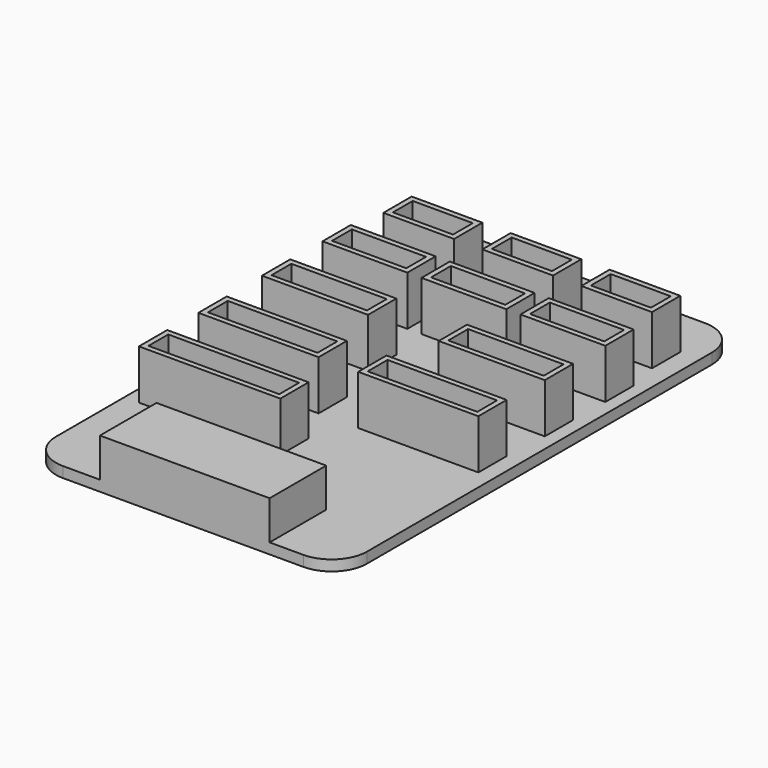
from build123d import *

# Parameters (mm, degrees)
F0_W         = 44
F0_H         = 71
F1_DEPTH     = 1.5
F2_R         = 5
F3_W         = 24
F3_H         = 10
F4_DEPTH     = 5.5
F5_W         = 10
F5_H         = 5
F5_W_2       = 12
F5_W_3       = 15
F5_W_4       = 17
F5_W_5       = 20
F6_DEPTH     = 7
F7_T         = 0.75
F7_T3_DEPTH  = 11.5
F7_T5_DEPTH  = 25.5
F7_T7_DEPTH  = 6.5
F7_T9_DEPTH  = 21.5
F7_T11_DEPTH = 6.5
F7_T13_DEPTH = 18.5
F7_T15_DEPTH = 18.5
F7_T17_DEPTH = 6.5
F7_T19_DEPTH = 16.5
F7_T21_DEPTH = 6.5
F7_T23_DEPTH = 13.5
F7_T25_DEPTH = 11.5
F7_T27_DEPTH = 6.5
F7_T29_DEPTH = 13.5
F7_T31_DEPTH = 16.5
F7_T33_DEPTH = 13.5
F7_T35_DEPTH = 11.5
F7_T37_DEPTH = 11.5


# Not quite as in the source:
# - a shell that OpenCascade refuses in one call is made with other operations: the cavity is built on its own and cut out


with BuildPart() as f1:
    # F0 (on Top) → F1 (new body)
    with BuildSketch(Plane.XY):
        with Locations((-0.4986094981, 2.3689430654)):
            Rectangle(F0_W, F0_H)
    extrude(amount=F1_DEPTH)

    # F2
    f2_edges = [f1.edges().sort_by_distance(p)[0] for p in [
        (-22.498609, 37.868943, 0.75),
        (-22.498609, -33.131057, 0.75),
        (21.501391, -33.131057, 0.75),
        (21.501391, 37.868943, 0.75),
    ]]
    fillet(f2_edges, radius=F2_R)

    # F3 (on face) → F4 (join)
    with BuildSketch(Plane.XY.offset(1.5)):
        with Locations((-0.276770547, -28.1310569346)):
            Rectangle(F3_W, F3_H)
    extrude(amount=F4_DEPTH)

    # F5 (on face) → F6 (join)
    with BuildSketch(Plane.XY.offset(1.5)):
        with Locations((-14.3074645847, 28.2659181952)):
            Rectangle(F5_W, F5_H)
        with Locations((-0.3074645847, 28.2659181952)):
            Rectangle(F5_W, F5_H)
        with Locations((13.6925354153, 28.2659181952)):
            Rectangle(F5_W, F5_H)
        with Locations((-14.3036200255, 18.7520762533)):
            Rectangle(F5_W_2, F5_H)
        with Locations((-0.3036200255, 18.7520762533)):
            Rectangle(F5_W_2, F5_H)
        with Locations((-12.8887149692, 8.1576090865)):
            Rectangle(F5_W_3, F5_H)
        with Locations((-11.8254707158, -3.1629925966)):
            Rectangle(F5_W_4, F5_H)
        with Locations((-10.4394350369, -13.5349402577)):
            Rectangle(F5_W_5, F5_H)
        with Locations((13.6963799745, 18.7520762533)):
            Rectangle(F5_W_2, F5_H)
        with Locations((12.1112850308, 8.1576090865)):
            Rectangle(F5_W_3, F5_H)
        with Locations((10.7745292842, -3.1629925966)):
            Rectangle(F5_W_4, F5_H)
    extrude(amount=F6_DEPTH)

    # F7: shell of thickness 0.75, made by hand


with BuildPart() as f7_core1:
    # F7_t2: copy of F1
    add(f1.part)

    # the walls: a layer under each face that stays
    f7_faces = [f7_core1.faces().sort_by_distance(p)[0] for p in [
        (-0.4986094981, -33.1310569346, 3.5),
        (-0.4986094981, 2.3689430654, 0),
        (-21.0341434041, -31.6665908405, 0.75),
        (-0.4986094981, 2.3689430654, 1.5),
        (-12.276770547, -28.1310569346, 4.25),
        (-0.276770547, -28.1310569346, 7),
        (11.723229453, -28.1310569346, 4.25),
        (20.0369244078, -31.6665908405, 0.75),
        (-22.4986094981, 2.3689430654, 0.75),
        (21.5013905019, 2.3689430654, 0.75),
        (-21.0341434041, 36.4044769713, 0.75),
        (20.0369244078, 36.4044769713, 0.75),
        (-0.4986094981, 37.8689430654, 0.75),
        (-0.276770547, -23.1310569346, 4.25),
        (-20.4394350369, -13.5349402577, 5),
        (-10.4394350369, -16.0349402577, 5),
        (-0.4394350369, -13.5349402577, 5),
        (-10.4394350369, -11.0349402577, 5),
        (-3.3254707158, -3.1629925966, 5),
        (-11.8254707158, -0.6629925966, 5),
        (-20.3254707158, -3.1629925966, 5),
        (-11.8254707158, -5.6629925966, 5),
        (19.2745292842, -3.1629925966, 5),
        (10.7745292842, -0.6629925966, 5),
        (2.2745292842, -3.1629925966, 5),
        (10.7745292842, -5.6629925966, 5),
        (-20.3887149692, 8.1576090865, 5),
        (-12.8887149692, 5.6576090865, 5),
        (-5.3887149692, 8.1576090865, 5),
        (-12.8887149692, 10.6576090865, 5),
        (-20.3036200255, 18.7520762533, 5),
        (-14.3036200255, 16.2520762533, 5),
        (-8.3036200255, 18.7520762533, 5),
        (-14.3036200255, 21.2520762533, 5),
        (-14.3074645847, 30.7659181952, 5),
        (-19.3074645847, 28.2659181952, 5),
        (-14.3074645847, 25.7659181952, 5),
        (-9.3074645847, 28.2659181952, 5),
        (-0.3036200255, 16.2520762533, 5),
        (5.6963799745, 18.7520762533, 5),
        (-0.3036200255, 21.2520762533, 5),
        (-6.3036200255, 18.7520762533, 5),
        (19.6112850308, 8.1576090865, 5),
        (12.1112850308, 10.6576090865, 5),
        (4.6112850308, 8.1576090865, 5),
        (12.1112850308, 5.6576090865, 5),
        (7.6963799745, 18.7520762533, 5),
        (13.6963799745, 16.2520762533, 5),
        (19.6963799745, 18.7520762533, 5),
        (13.6963799745, 21.2520762533, 5),
        (-0.3074645847, 25.7659181952, 5),
        (4.6925354153, 28.2659181952, 5),
        (-0.3074645847, 30.7659181952, 5),
        (-5.3074645847, 28.2659181952, 5),
        (13.6925354153, 30.7659181952, 5),
        (8.6925354153, 28.2659181952, 5),
        (13.6925354153, 25.7659181952, 5),
        (18.6925354153, 28.2659181952, 5),
    ]]
    thicken(f7_faces, amount=-F7_T, mode=Mode.SUBTRACT)

    # F7_s4 → F7_t3 (cut)
    with BuildSketch(Plane.XZ.offset(22.3810569346)):
        Polygon((-12.284270547, 1.5075), (-12.276770547, 0.75), (-11.526770547, 0.75), (-11.526770547, 1.5), align=None)
        Polygon((11.730729453, 1.5075), (11.723229453, 0.75), (10.973229453, 0.75), (10.973229453, 1.5), align=None)
    extrude(amount=F7_T3_DEPTH, mode=Mode.SUBTRACT)

    # F7_s6 → F7_t5 (cut)
    with BuildSketch(Plane.YZ.offset(-13.026770547)):
        Polygon((-23.1235569346, 1.5075), (-23.1310569346, 0.75), (-23.8810569346, 0.75), (-23.8810569346, 1.5), align=None)
    extrude(amount=F7_T5_DEPTH, mode=Mode.SUBTRACT)

    # F7_s8 → F7_t7 (cut)
    with BuildSketch(Plane.XZ.offset(10.2849402577)):
        Polygon((-20.4469350369, 1.5075), (-20.4394350369, 0.75), (-19.6894350369, 0.75), (-19.6894350369, 1.5), align=None)
        Polygon((-0.4319350369, 1.5075), (-0.4394350369, 0.75), (-1.1894350369, 0.75), (-1.1894350369, 1.5), align=None)
    extrude(amount=F7_T7_DEPTH, mode=Mode.SUBTRACT)

    # F7_s10 → F7_t9 (cut)
    with BuildSketch(Plane.YZ.offset(-21.1894350369)):
        Polygon((-16.0424402577, 1.5075), (-16.0349402577, 0.75), (-15.2849402577, 0.75), (-15.2849402577, 1.5), align=None)
        Polygon((-11.0274402577, 1.5075), (-11.0349402577, 0.75), (-11.7849402577, 0.75), (-11.7849402577, 1.5), align=None)
    extrude(amount=F7_T9_DEPTH, mode=Mode.SUBTRACT)

    # F7_s12 → F7_t11 (cut)
    with BuildSketch(Plane.XZ.offset(-0.0870074034)):
        Polygon((-3.3179707158, 1.5075), (-3.3254707158, 0.75), (-4.0754707158, 0.75), (-4.0754707158, 1.5), align=None)
        Polygon((-20.3329707158, 1.5075), (-20.3254707158, 0.75), (-19.5754707158, 0.75), (-19.5754707158, 1.5), align=None)
        Polygon((19.2820292842, 1.5075), (19.2745292842, 0.75), (18.5245292842, 0.75), (18.5245292842, 1.5), align=None)
        Polygon((2.2670292842, 1.5075), (2.2745292842, 0.75), (3.0245292842, 0.75), (3.0245292842, 1.5), align=None)
    extrude(amount=F7_T11_DEPTH, mode=Mode.SUBTRACT)

    # F7_s14 → F7_t13 (cut)
    with BuildSketch(Plane.YZ.offset(-21.0754707158)):
        Polygon((-0.6554925966, 1.5075), (-0.6629925966, 0.75), (-1.4129925966, 0.75), (-1.4129925966, 1.5), align=None)
        Polygon((-5.6704925966, 1.5075), (-5.6629925966, 0.75), (-4.9129925966, 0.75), (-4.9129925966, 1.5), align=None)
    extrude(amount=F7_T13_DEPTH, mode=Mode.SUBTRACT)

    # F7_s16 → F7_t15 (cut)
    with BuildSketch(Plane.YZ.offset(1.5245292842)):
        Polygon((-0.6554925966, 1.5075), (-0.6629925966, 0.75), (-1.4129925966, 0.75), (-1.4129925966, 1.5), align=None)
        Polygon((-5.6704925966, 1.5075), (-5.6629925966, 0.75), (-4.9129925966, 0.75), (-4.9129925966, 1.5), align=None)
    extrude(amount=F7_T15_DEPTH, mode=Mode.SUBTRACT)

    # F7_s18 → F7_t17 (cut)
    with BuildSketch(Plane.XZ.offset(-11.4076090865)):
        Polygon((-20.3962149692, 1.5075), (-20.3887149692, 0.75), (-19.6387149692, 0.75), (-19.6387149692, 1.5), align=None)
        Polygon((-5.3812149692, 1.5075), (-5.3887149692, 0.75), (-6.1387149692, 0.75), (-6.1387149692, 1.5), align=None)
        Polygon((19.6187850308, 1.5075), (19.6112850308, 0.75), (18.8612850308, 0.75), (18.8612850308, 1.5), align=None)
        Polygon((4.6037850308, 1.5075), (4.6112850308, 0.75), (5.3612850308, 0.75), (5.3612850308, 1.5), align=None)
    extrude(amount=F7_T17_DEPTH, mode=Mode.SUBTRACT)

    # F7_s20 → F7_t19 (cut)
    with BuildSketch(Plane.YZ.offset(-21.1387149692)):
        Polygon((5.6501090865, 1.5075), (5.6576090865, 0.75), (6.4076090865, 0.75), (6.4076090865, 1.5), align=None)
        Polygon((10.6651090865, 1.5075), (10.6576090865, 0.75), (9.9076090865, 0.75), (9.9076090865, 1.5), align=None)
    extrude(amount=F7_T19_DEPTH, mode=Mode.SUBTRACT)

    # F7_s22 → F7_t21 (cut)
    with BuildSketch(Plane.XZ.offset(-22.0020762533)):
        Polygon((-20.3111200255, 1.5075), (-20.3036200255, 0.75), (-19.5536200255, 0.75), (-19.5536200255, 1.5), align=None)
        Polygon((-8.2961200255, 1.5075), (-8.3036200255, 0.75), (-9.0536200255, 0.75), (-9.0536200255, 1.5), align=None)
        Polygon((5.7038799745, 1.5075), (5.6963799745, 0.75), (4.9463799745, 0.75), (4.9463799745, 1.5), align=None)
        Polygon((-6.3111200255, 1.5075), (-6.3036200255, 0.75), (-5.5536200255, 0.75), (-5.5536200255, 1.5), align=None)
        Polygon((7.6888799745, 1.5075), (7.6963799745, 0.75), (8.4463799745, 0.75), (8.4463799745, 1.5), align=None)
        Polygon((19.7038799745, 1.5075), (19.6963799745, 0.75), (18.9463799745, 0.75), (18.9463799745, 1.5), align=None)
    extrude(amount=F7_T21_DEPTH, mode=Mode.SUBTRACT)

    # F7_s24 → F7_t23 (cut)
    with BuildSketch(Plane.YZ.offset(-21.0536200255)):
        Polygon((16.2445762533, 1.5075), (16.2520762533, 0.75), (17.0020762533, 0.75), (17.0020762533, 1.5), align=None)
        Polygon((21.2595762533, 1.5075), (21.2520762533, 0.75), (20.5020762533, 0.75), (20.5020762533, 1.5), align=None)
    extrude(amount=F7_T23_DEPTH, mode=Mode.SUBTRACT)

    # F7_s26 → F7_t25 (cut)
    with BuildSketch(Plane.YZ.offset(-20.0574645847)):
        Polygon((30.7734181952, 1.5075), (30.7659181952, 0.75), (30.0159181952, 0.75), (30.0159181952, 1.5), align=None)
        Polygon((25.7584181952, 1.5075), (25.7659181952, 0.75), (26.5159181952, 0.75), (26.5159181952, 1.5), align=None)
    extrude(amount=F7_T25_DEPTH, mode=Mode.SUBTRACT)

    # F7_s28 → F7_t27 (cut)
    with BuildSketch(Plane.XZ.offset(-31.5159181952)):
        Polygon((-19.3149645847, 1.5075), (-19.3074645847, 0.75), (-18.5574645847, 0.75), (-18.5574645847, 1.5), align=None)
        Polygon((-9.2999645847, 1.5075), (-9.3074645847, 0.75), (-10.0574645847, 0.75), (-10.0574645847, 1.5), align=None)
        Polygon((4.7000354153, 1.5075), (4.6925354153, 0.75), (3.9425354153, 0.75), (3.9425354153, 1.5), align=None)
        Polygon((-5.3149645847, 1.5075), (-5.3074645847, 0.75), (-4.5574645847, 0.75), (-4.5574645847, 1.5), align=None)
        Polygon((8.6850354153, 1.5075), (8.6925354153, 0.75), (9.4425354153, 0.75), (9.4425354153, 1.5), align=None)
        Polygon((18.7000354153, 1.5075), (18.6925354153, 0.75), (17.9425354153, 0.75), (17.9425354153, 1.5), align=None)
    extrude(amount=F7_T27_DEPTH, mode=Mode.SUBTRACT)

    # F7_s30 → F7_t29 (cut)
    with BuildSketch(Plane.YZ.offset(-7.0536200255)):
        Polygon((16.2445762533, 1.5075), (16.2520762533, 0.75), (17.0020762533, 0.75), (17.0020762533, 1.5), align=None)
        Polygon((21.2595762533, 1.5075), (21.2520762533, 0.75), (20.5020762533, 0.75), (20.5020762533, 1.5), align=None)
    extrude(amount=F7_T29_DEPTH, mode=Mode.SUBTRACT)

    # F7_s32 → F7_t31 (cut)
    with BuildSketch(Plane.YZ.offset(3.8612850308)):
        Polygon((10.6651090865, 1.5075), (10.6576090865, 0.75), (9.9076090865, 0.75), (9.9076090865, 1.5), align=None)
        Polygon((5.6501090865, 1.5075), (5.6576090865, 0.75), (6.4076090865, 0.75), (6.4076090865, 1.5), align=None)
    extrude(amount=F7_T31_DEPTH, mode=Mode.SUBTRACT)

    # F7_s34 → F7_t33 (cut)
    with BuildSketch(Plane.YZ.offset(6.9463799745)):
        Polygon((16.2445762533, 1.5075), (16.2520762533, 0.75), (17.0020762533, 0.75), (17.0020762533, 1.5), align=None)
        Polygon((21.2595762533, 1.5075), (21.2520762533, 0.75), (20.5020762533, 0.75), (20.5020762533, 1.5), align=None)
    extrude(amount=F7_T33_DEPTH, mode=Mode.SUBTRACT)

    # F7_s36 → F7_t35 (cut)
    with BuildSketch(Plane.YZ.offset(-6.0574645847)):
        Polygon((25.7584181952, 1.5075), (25.7659181952, 0.75), (26.5159181952, 0.75), (26.5159181952, 1.5), align=None)
        Polygon((30.7734181952, 1.5075), (30.7659181952, 0.75), (30.0159181952, 0.75), (30.0159181952, 1.5), align=None)
    extrude(amount=F7_T35_DEPTH, mode=Mode.SUBTRACT)

    # F7_s38 → F7_t37 (cut)
    with BuildSketch(Plane.YZ.offset(7.9425354153)):
        Polygon((30.7734181952, 1.5075), (30.7659181952, 0.75), (30.0159181952, 0.75), (30.0159181952, 1.5), align=None)
        Polygon((25.7584181952, 1.5075), (25.7659181952, 0.75), (26.5159181952, 0.75), (26.5159181952, 1.5), align=None)
    extrude(amount=F7_T37_DEPTH, mode=Mode.SUBTRACT)


with BuildPart() as f1_1:
    add(f1.part)

    # what is left inside the walls is the cavity
    f7_cavity = [f7_core1.part.solids().sort_by_distance(p)[0] for p in [
        (-0.276771, -29.547724, 6.2425),
        (-7.356102, -15.27744, 4.625),
        (-9.242137, -1.420493, 4.625),
        (13.357863, -1.420493, 4.625),
        (-10.638715, 9.900109, 4.625),
        (-12.55362, 17.009576, 4.625),
        (-12.890798, 30.008418, 4.625),
        (1.44638, 17.009576, 4.625),
        (14.361285, 6.415109, 4.625),
        (15.44638, 17.009576, 4.625),
        (1.109202, 26.523418, 4.625),
        (15.109202, 30.008418, 4.625),
    ]]
    add(f7_cavity, mode=Mode.SUBTRACT)


solid = f1_1.part
